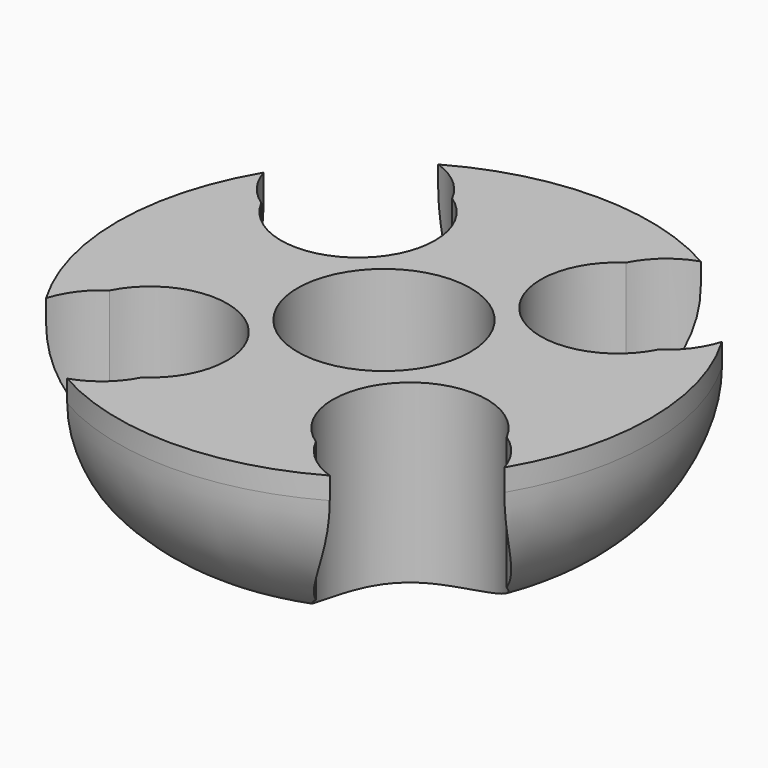
from build123d import *

# Parameters (mm, degrees)
F0_R           = 12.1
F0_R_2         = 3.925
F1_DEPTH       = 8
F2_D           = 5
F2_DEPTH       = 12
F2_CBORE_D     = 7
F2_CBORE_DEPTH = 9
F2_TIP         = 1.5021515476
F3_R           = 7


# Not quite as in the source:
# - a feature names something its author has since deleted; it is built from what else it names


with BuildPart() as f1:
    # F0 (on Top) → F1 (new body)
    with BuildSketch(Plane.XY):
        Circle(F0_R)
        with BuildLine():
            Line((-8.3705968588, -6.0454343887), (-7.2080156238, -4.737418765))
            ThreePointArc((-7.2080156238, -4.737418765), (-4.737418765, -4.5919843762), (-4.5919843762, -7.062581235))
            Line((-4.5919843762, -7.062581235), (-5.7545656113, -8.3705968588))
            ThreePointArc((-5.7545656113, -8.3705968588), (-8.22516247, -8.5160312475), (-8.3705968588, -6.0454343887))
        make_face(mode=Mode.SUBTRACT)
        with BuildLine():
            ThreePointArc((4.5919843762, -7.062581235), (4.737418765, -4.5919843762), (7.2080156238, -4.737418765))
            Line((7.2080156238, -4.737418765), (8.3705968588, -6.0454343887))
            ThreePointArc((8.3705968588, -6.0454343887), (8.22516247, -8.5160312475), (5.7545656113, -8.3705968588))
            Line((5.7545656113, -8.3705968588), (4.5919843762, -7.062581235))
        make_face(mode=Mode.SUBTRACT)
        with BuildLine():
            ThreePointArc((-8.3705968588, 6.0454343887), (-8.22516247, 8.5160312475), (-5.7545656113, 8.3705968588))
            Line((-5.7545656113, 8.3705968588), (-4.5919843762, 7.062581235))
            ThreePointArc((-4.5919843762, 7.062581235), (-4.737418765, 4.5919843762), (-7.2080156238, 4.737418765))
            Line((-7.2080156238, 4.737418765), (-8.3705968588, 6.0454343887))
        make_face(mode=Mode.SUBTRACT)
        Circle(F0_R_2, mode=Mode.SUBTRACT)
        with BuildLine():
            Line((8.3705968588, 6.0454343887), (7.2080156238, 4.737418765))
            ThreePointArc((7.2080156238, 4.737418765), (4.737418765, 4.5919843762), (4.5919843762, 7.062581235))
            Line((4.5919843762, 7.062581235), (5.7545656113, 8.3705968588))
            ThreePointArc((5.7545656113, 8.3705968588), (8.22516247, 8.5160312475), (8.3705968588, 6.0454343887))
        make_face(mode=Mode.SUBTRACT)
    extrude(amount=-F1_DEPTH)

    # F2
    with Locations(Plane.XY):
        with Locations((-5.9, 5.9), (-7.062581235, 7.2080156238), (-7.062581235, -7.2080156238), (7.062581235, -7.2080156238), (5.9, -5.9), (5.9, 5.9), (7.062581235, 7.2080156238), (-5.9, -5.9)):
            CounterBoreHole(F2_D / 2, F2_CBORE_D / 2, F2_CBORE_DEPTH, depth=F2_DEPTH)
            with Locations((0, 0, -(F2_DEPTH + F2_TIP / 2))):  # 118° drill point
                Cone(0, F2_D / 2, F2_TIP, mode=Mode.SUBTRACT)

    # F3
    f3_edges = [f1.edges().sort_by_distance(p)[0] for p in [
        (12.1, 0, -8),
        (0, 12.1, -8),
        (-12.1, 0, -8),
        (0, -12.1, -8),
    ]]
    fillet(f3_edges, radius=F3_R)


solid = f1.part
